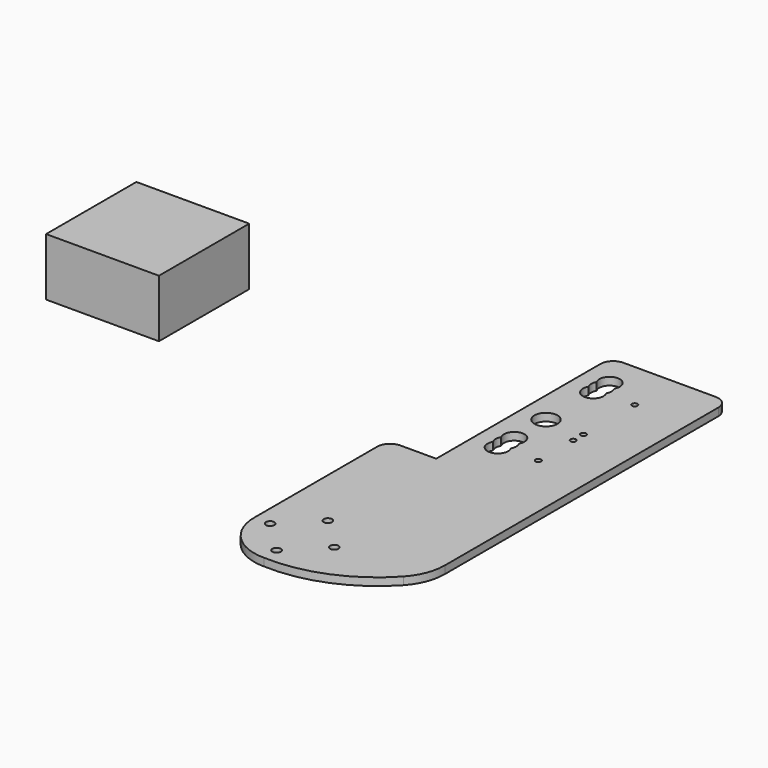
from build123d import *

# Parameters (mm, degrees)
F0_R     = 3.25
F0_R_2   = 2.15
F0_R_3   = 9
F1_DEPTH = 6
F0_W     = 88
F0_H     = 88
F2_DEPTH = 45


# Not quite as in the source:
# - a feature names something its author has since deleted; it is built from what else it names


with BuildPart() as f1:
    # F0 (on Top) → F1 (new body)
    with BuildSketch(Plane.XY):
        with BuildLine():
            Line((-37.5, 29.9842730165), (-37.5, 0))
            ThreePointArc((-37.5, 0), (-26.5165042945, -26.5165042945), (0, -37.5))
            ThreePointArc((0, -37.5), (44.6548482199, -29.7050919513), (81.8756191651, -3.8317413512))
            ThreePointArc((81.8756191651, -3.8317413512), (89.7493272866, 8.7403920196), (92.5, 23.3173470068))
            Line((92.5, 23.3173470068), (92.5, 75.5242775083))
            Line((92.5, 75.5242775083), (92.5, 130))
            Line((92.5, 130), (92.5, 276))
            Line((92.5, 276), (92.5, 286.8150174618))
            Line((92.5, 286.8150174618), (92.5, 290))
            ThreePointArc((92.5, 290), (89.5710678119, 297.0710678119), (82.5, 300))
            Line((82.5, 300), (10.5, 300))
            ThreePointArc((10.5, 300), (3.4289321881, 297.0710678119), (0.5, 290))
            Line((0.5, 290), (0.5, 160))
            Line((0.5, 160), (0.5, 143.811336026))
            Line((0.5, 143.811336026), (0.5, 130))
            Line((0.5, 130), (-27.5, 130))
            ThreePointArc((-27.5, 130), (-34.5710678119, 127.0710678119), (-37.5, 120))
            Line((-37.5, 120), (-37.5, 29.9842730165))
        make_face()
        with Locations((-25, 0)):
            Circle(F0_R, mode=Mode.SUBTRACT)
        with Locations((0, -25)):
            Circle(F0_R, mode=Mode.SUBTRACT)
        with Locations((25, 0)):
            Circle(F0_R, mode=Mode.SUBTRACT)
        with Locations((0, 25)):
            Circle(F0_R, mode=Mode.SUBTRACT)
        with BuildLine():
            ThreePointArc((27.4282032303, 169), (28.2274066103, 167.0705523608), (28.5, 165))
            ThreePointArc((28.5, 165), (18.4294476392, 157.2725933897), (13.5717967697, 169))
            ThreePointArc((13.5717967697, 169), (12.5, 173), (13.5717967697, 177))
            ThreePointArc((13.5717967697, 177), (18.4294476392, 188.7274066103), (28.5, 181))
            ThreePointArc((28.5, 181), (28.2274066103, 178.9294476392), (27.4282032303, 177))
            ThreePointArc((27.4282032303, 177), (28.2274066103, 175.0705523608), (28.5, 173))
            ThreePointArc((28.5, 173), (28.2274066103, 170.9294476392), (27.4282032303, 169))
        make_face(mode=Mode.SUBTRACT)
        with Locations((50.5, 167)):
            Circle(F0_R_2, mode=Mode.SUBTRACT)
        with Locations((20.5, 212)):
            Circle(F0_R_3, mode=Mode.SUBTRACT)
        with Locations((50.5, 201)):
            Circle(F0_R_2, mode=Mode.SUBTRACT)
        with Locations((50.5, 211)):
            Circle(F0_R_2, mode=Mode.SUBTRACT)
        with BuildLine():
            ThreePointArc((27.4282032303, 262), (28.2274066103, 260.0705523608), (28.5, 258))
            ThreePointArc((28.5, 258), (18.4294476392, 250.2725933897), (13.5717967697, 262))
            ThreePointArc((13.5717967697, 262), (12.5, 266), (13.5717967697, 270))
            ThreePointArc((13.5717967697, 270), (18.4294476392, 281.7274066103), (28.5, 274))
            ThreePointArc((28.5, 274), (28.2274066103, 271.9294476392), (27.4282032303, 270))
            ThreePointArc((27.4282032303, 270), (28.2274066103, 268.0705523608), (28.5, 266))
            ThreePointArc((28.5, 266), (28.2274066103, 263.9294476392), (27.4282032303, 262))
        make_face(mode=Mode.SUBTRACT)
        with Locations((50.5, 261)):
            Circle(F0_R_2, mode=Mode.SUBTRACT)
    extrude(amount=F1_DEPTH)


with BuildPart() as f2:
    # F0 (on Top) → F2 (new body)
    with BuildSketch(Plane.XY):
        with Locations((-279.2910335064, 198.4254124165)):
            Rectangle(F0_W, F0_H)
    extrude(amount=F2_DEPTH)


solid = Compound([f1.part, f2.part])
